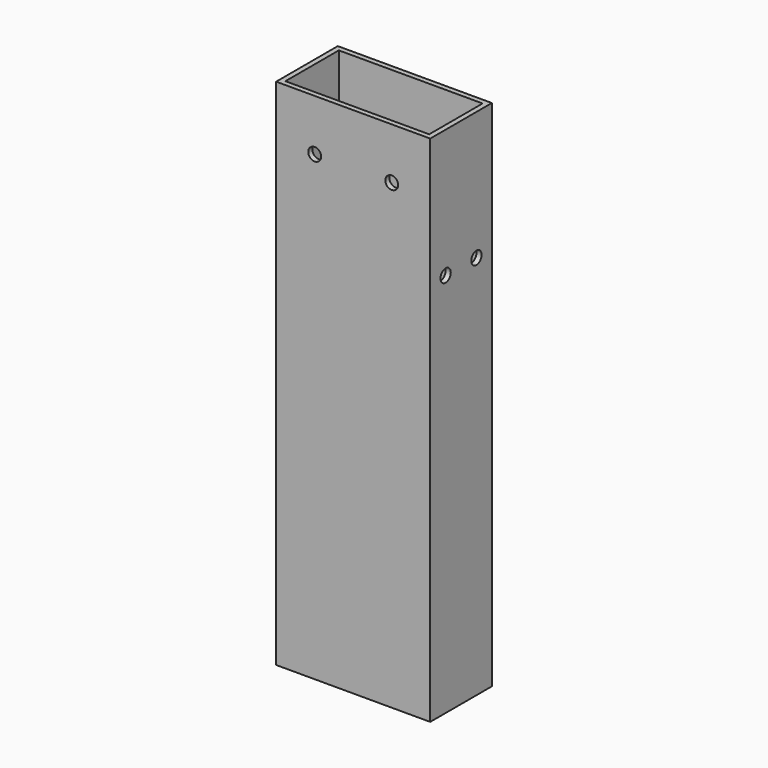
from build123d import *

# Parameters (mm, degrees)
F0_W       = 76.2
F0_H       = 38.1
F1_DEPTH   = 254
F2_T       = -2.54
F5_D       = 6.35
F5_ON_F4_D = 6.35
F7_D       = 12.7


with BuildPart() as f1:
    # F0 (on Top) → F1 (new body)
    with BuildSketch(Plane.XY):
        Rectangle(F0_W, F0_H)
    extrude(amount=F1_DEPTH)

    # F2
    f2_openings = [f1.faces().sort_by_distance(p)[0] for p in [
        (0, 0, 254),
    ]]
    offset(amount=F2_T, openings=f2_openings)

    # F5 (through all)
    with Locations(Plane(origin=(-38.1, 0, 0), x_dir=(0, -1, 0), z_dir=(-1, 0, 0))):
        with Locations((-9.525, 190.5), (9.525, 190.5)):
            Hole(F5_D / 2)

    # F5 on F4 (through all)
    with Locations(Plane.XZ.offset(19.05)):
        with Locations((-19.05, 228.6), (19.05, 228.6)):
            Hole(F5_ON_F4_D / 2)

    # F7 (through all)
    with Locations(Plane(origin=(0, 0, 0), x_dir=(1, 0, 0), z_dir=(0, 0, -1))):
        with Locations((0, 0)):
            Hole(F7_D / 2)


solid = f1.part
